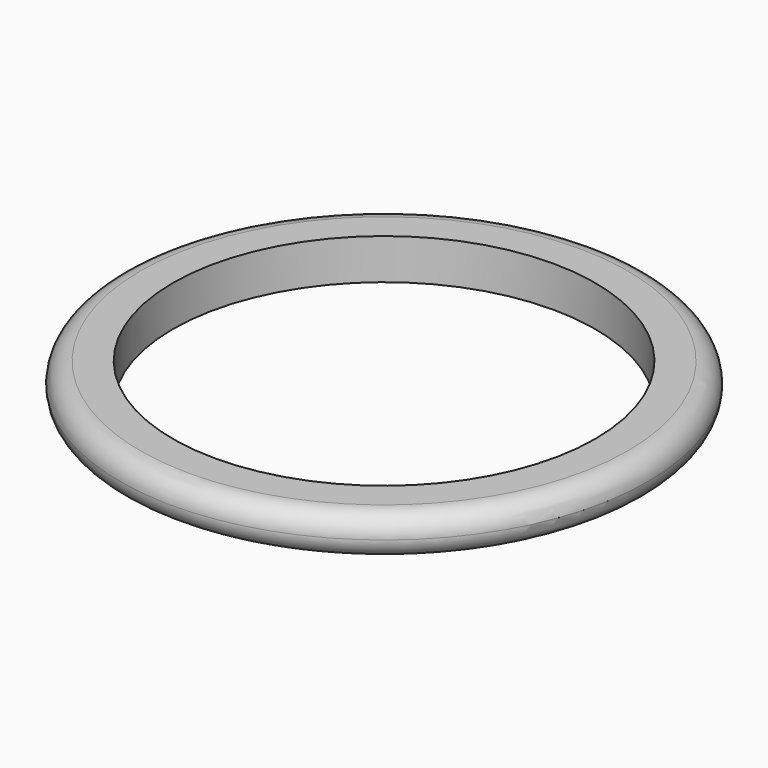
from build123d import *

# Parameters (mm, degrees)
F0_R     = 32.5
F0_R_2   = 26
F1_DEPTH = 5
F2_R     = 2.49999


# Not quite as in the source:
# - a fillet or chamfer is up to 0.001 mm smaller than in the source, because OpenCascade refuses the exact size


with BuildPart() as f1:
    # F0 (on Top) → F1 (new body)
    with BuildSketch(Plane.XY):
        Circle(F0_R)
        Circle(F0_R_2, mode=Mode.SUBTRACT)
    extrude(amount=F1_DEPTH)

    # F2 (radius 2.5 in the source; OpenCascade refuses exactly that, so slightly less here)
    f2_edges = [f1.edges().sort_by_distance(p)[0] for p in [
        (32.5, 0, 2.5),
        (-32.5, 0, 0),
        (-32.5, 0, 5),
    ]]
    fillet(f2_edges, radius=F2_R)


solid = f1.part
